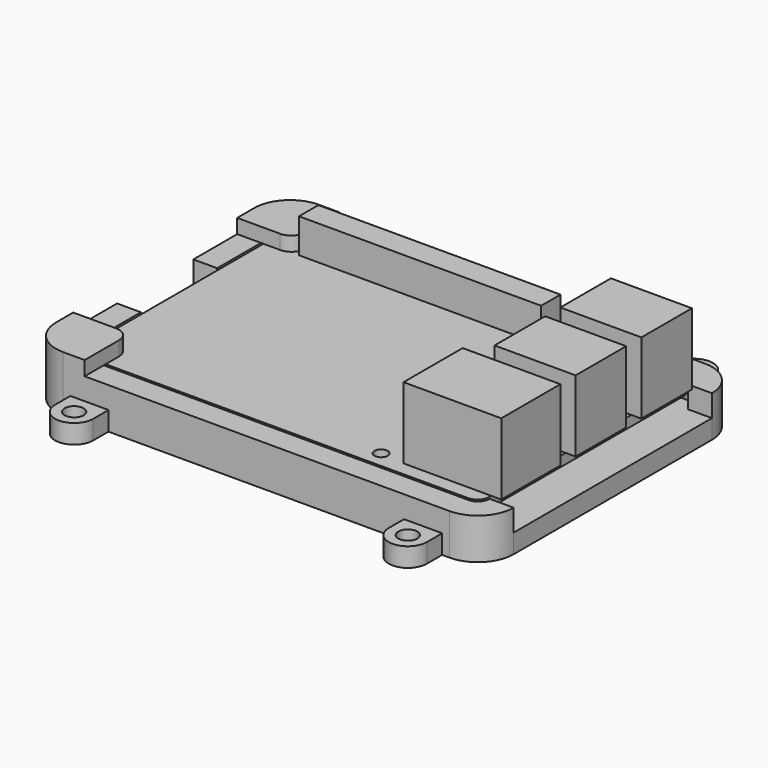
from build123d import *

# Parameters (mm, degrees)
F0_R      = 1.4
F1_DEPTH  = 2.1
F2_W      = 50.8
F2_H      = 5.08
F3_DEPTH  = 7.2
F4_W      = 17
F4_H      = 13.25
F4_W_2    = 20.5
F4_H_2    = 15.5
F5_DEPTH  = 15
F8_DEPTH  = 4.6
F10_DEPTH = 2.5
F12_DEPTH = 4
F13_W     = 32.5408354402
F13_H     = 52
F14_DEPTH = 4.6
F16_DEPTH = 3
F17_R     = 2
F18_DEPTH = 4


with BuildPart() as f1:
    # F0 (on Top) → F1 (new body)
    with BuildSketch(Plane.XY):
        with BuildLine():
            Line((40, 28), (-40, 28))
            ThreePointArc((-40, 28), (-41.767766953, 27.267766953), (-42.5, 25.5))
            Line((-42.5, 25.5), (-42.5, -25.5))
            ThreePointArc((-42.5, -25.5), (-41.767766953, -27.267766953), (-40, -28))
            Line((-40, -28), (40, -28))
            ThreePointArc((40, -28), (41.767766953, -27.267766953), (42.5, -25.5))
            Line((42.5, -25.5), (42.5, 25.5))
            ThreePointArc((42.5, 25.5), (41.767766953, 27.267766953), (40, 28))
        make_face()
        with Locations((-39, -24.5)):
            Circle(F0_R, mode=Mode.SUBTRACT)
        with Locations((19, -24.5)):
            Circle(F0_R, mode=Mode.SUBTRACT)
        with Locations((-39, 24.5)):
            Circle(F0_R, mode=Mode.SUBTRACT)
        with Locations((19, 24.5)):
            Circle(F0_R, mode=Mode.SUBTRACT)
    extrude(amount=F1_DEPTH)

    # F2 (on face) → F3 (join)
    with BuildSketch(Plane.XY.offset(2.1)):
        with Locations((-10, 24.5)):
            Rectangle(F2_W, F2_H)
    extrude(amount=F3_DEPTH)

    # F4 (on face) → F5 (join)
    with BuildSketch(Plane.XY.offset(2.1)):
        with Locations((36.1, 18.375)):
            Rectangle(F4_W, F4_H)
        with Locations((36.1, 1.125)):
            Rectangle(F4_W, F4_H)
        with Locations((34.35, -17.25)):
            Rectangle(F4_W_2, F4_H_2)
    extrude(amount=F5_DEPTH)


with BuildPart() as f8:
    # F7 (on offset) → F8 (new body, through all)
    with BuildSketch(Plane.XY.offset(-2.5)):
        with BuildLine():
            ThreePointArc((-43, 26), (-42.267766953, 27.767766953), (-40.5, 28.5))
            Line((-40.5, 28.5), (40.5, 28.5))
            ThreePointArc((40.5, 28.5), (42.267766953, 27.767766953), (43, 26))
            Line((43, 26), (43, -26))
            ThreePointArc((43, -26), (42.267766953, -27.767766953), (40.5, -28.5))
            Line((40.5, -28.5), (-40.5, -28.5))
            ThreePointArc((-40.5, -28.5), (-42.267766953, -27.767766953), (-43, -26))
            Line((-43, -26), (-43, -10))
            Line((-43, -10), (-48, -10))
            Line((-48, -10), (-48, -26))
            ThreePointArc((-48, -26), (-45.8033008589, -31.3033008589), (-40.5, -33.5))
            Line((-40.5, -33.5), (40.5, -33.5))
            ThreePointArc((40.5, -33.5), (45.8033008589, -31.3033008589), (48, -26))
            Line((48, -26), (48, 26))
            ThreePointArc((48, 26), (45.8033008589, 31.3033008589), (40.5, 33.5))
            Line((40.5, 33.5), (-40.5, 33.5))
            ThreePointArc((-40.5, 33.5), (-45.8033008589, 31.3033008589), (-48, 26))
            Line((-48, 26), (-48, 10))
            Line((-48, 10), (-43, 10))
            Line((-43, 10), (-43, 26))
        make_face()
    extrude(amount=F8_DEPTH)

    # F9 (on offset) → F10 (join, through all)
    with BuildSketch(Plane.XY.offset(-2.5)):
        with BuildLine():
            Line((22, -28.5), (22, -24.5))
            ThreePointArc((22, -24.5), (19, -21.5), (16, -24.5))
            Line((16, -24.5), (16, -28.5))
            Line((16, -28.5), (22, -28.5))
        make_face()
        with BuildLine():
            Line((22, 28.5), (16, 28.5))
            Line((16, 28.5), (16, 24.5))
            ThreePointArc((16, 24.5), (19, 21.5), (22, 24.5))
            Line((22, 24.5), (22, 28.5))
        make_face()
        with BuildLine():
            Line((-43, 21.5), (-39, 21.5))
            ThreePointArc((-39, 21.5), (-36.8786796564, 22.3786796564), (-36, 24.5))
            Line((-36, 24.5), (-36, 28.5))
            Line((-36, 28.5), (-43, 28.5))
            Line((-43, 28.5), (-43, 21.5))
        make_face()
        with BuildLine():
            ThreePointArc((-36, -24.5), (-36.8786796564, -22.3786796564), (-39, -21.5))
            Line((-39, -21.5), (-43, -21.5))
            Line((-43, -21.5), (-43, -28.5))
            Line((-43, -28.5), (-36, -28.5))
            Line((-36, -28.5), (-36, -24.5))
        make_face()
    extrude(amount=F10_DEPTH)

    # F11 (on offset) → F12 (join)
    with BuildSketch(Plane.XY.offset(-2.5)):
        with BuildLine():
            ThreePointArc((-48, -26), (-45.8033008589, -31.3033008589), (-40.5, -33.5))
            Line((-40.5, -33.5), (40.5, -33.5))
            ThreePointArc((40.5, -33.5), (45.8033008589, -31.3033008589), (48, -26))
            Line((48, -26), (48, 26))
            ThreePointArc((48, 26), (45.8033008589, 31.3033008589), (40.5, 33.5))
            Line((40.5, 33.5), (-40.5, 33.5))
            ThreePointArc((-40.5, 33.5), (-45.8033008589, 31.3033008589), (-48, 26))
            Line((-48, 26), (-48, -26))
        make_face()
    extrude(amount=-F12_DEPTH)

    # F13 (on face) → F14 (cut, through all)
    with BuildSketch(Plane.XY.offset(2.1)):
        with Locations((59.2704177201, 0)):
            Rectangle(F13_W, F13_H)
    extrude(amount=-F14_DEPTH, mode=Mode.SUBTRACT)

    # F15 (on face) → F16 (join)
    with BuildSketch(Plane.XY.offset(2.1)):
        with BuildLine():
            Line((-36, 33.5), (-40.5, 33.5))
            ThreePointArc((-40.5, 33.5), (-45.8033008589, 31.3033008589), (-48, 26))
            Line((-48, 26), (-48, 21.5))
            Line((-48, 21.5), (-39, 21.5))
            ThreePointArc((-39, 21.5), (-36.8786796564, 22.3786796564), (-36, 24.5))
            Line((-36, 24.5), (-36, 33.5))
        make_face()
        with BuildLine():
            ThreePointArc((-36, -24.5), (-36.8786796564, -22.3786796564), (-39, -21.5))
            Line((-39, -21.5), (-48, -21.5))
            Line((-48, -21.5), (-48, -26))
            ThreePointArc((-48, -26), (-45.8033008589, -31.3033008589), (-40.5, -33.5))
            Line((-40.5, -33.5), (-36, -33.5))
            Line((-36, -33.5), (-36, -24.5))
        make_face()
    extrude(amount=F16_DEPTH)

    # F17 (on face) → F18 (join)
    with BuildSketch(Plane(origin=(0, 0, -6.5), x_dir=(1, 0, 0), z_dir=(0, 0, -1))):
        with BuildLine():
            Line((-39, -33.5), (-39, -37.5))
            ThreePointArc((-39, -37.5), (-35, -41.5), (-31, -37.5))
            Line((-31, -37.5), (-31, -33.5))
            Line((-31, -33.5), (-39, -33.5))
        make_face()
        with Locations((-35, -37.5)):
            Circle(F17_R, mode=Mode.SUBTRACT)
        with BuildLine():
            Line((39, -33.5), (31, -33.5))
            Line((31, -33.5), (31, -37.5))
            ThreePointArc((31, -37.5), (35, -41.5), (39, -37.5))
            Line((39, -37.5), (39, -33.5))
        make_face()
        with Locations((35, -37.5)):
            Circle(F17_R, mode=Mode.SUBTRACT)
        with BuildLine():
            Line((31, 37.5), (31, 33.5))
            Line((31, 33.5), (39, 33.5))
            Line((39, 33.5), (39, 37.5))
            ThreePointArc((39, 37.5), (35, 41.5), (31, 37.5))
        make_face()
        with Locations((35, 37.5)):
            Circle(F17_R, mode=Mode.SUBTRACT)
        with BuildLine():
            ThreePointArc((-31, 37.5), (-35, 41.5), (-39, 37.5))
            Line((-39, 37.5), (-39, 33.5))
            Line((-39, 33.5), (-31, 33.5))
            Line((-31, 33.5), (-31, 37.5))
        make_face()
        with Locations((-35, 37.5)):
            Circle(F17_R, mode=Mode.SUBTRACT)
    extrude(amount=-F18_DEPTH)


solid = Compound([f1.part, f8.part])
